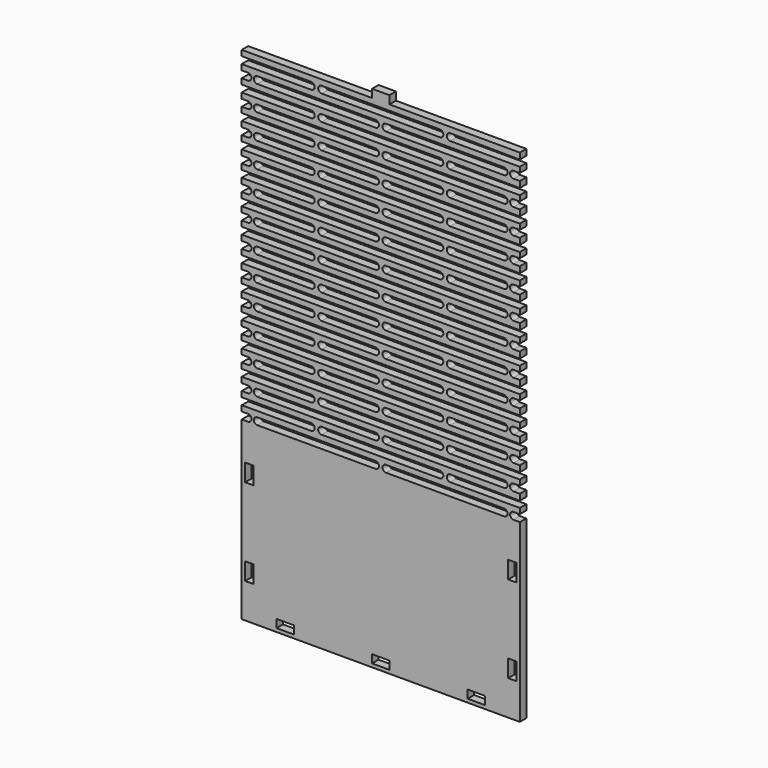
from build123d import *

# Parameters (mm, degrees)
F0_W     = 101.6
F0_H     = 63.5
F0_W_2   = 2.9718
F0_H_2   = 6.35
F0_W_3   = 6.35
F0_H_3   = 2.9718
F1_DEPTH = 2.9718


with BuildPart() as f1:
    # F0 (on Front) → F1 (new body)
    with BuildSketch(Plane.XZ):
        with Locations((0.0203015033, 4.5659675)):
            Rectangle(F0_W, F0_H)
        with Locations((-48.0237984967, -11.3090325)):
            Rectangle(F0_W_2, F0_H_2, mode=Mode.SUBTRACT)
        with Locations((-34.9046984967, -24.4281325)):
            Rectangle(F0_W_3, F0_H_3, mode=Mode.SUBTRACT)
        with Locations((0.0203015033, -24.4281325)):
            Rectangle(F0_W_3, F0_H_3, mode=Mode.SUBTRACT)
        with Locations((-48.0237984967, 20.4409675)):
            Rectangle(F0_W_2, F0_H_2, mode=Mode.SUBTRACT)
        with Locations((34.9453015033, -24.4281325)):
            Rectangle(F0_W_3, F0_H_3, mode=Mode.SUBTRACT)
        with Locations((48.0644015033, -11.3090325)):
            Rectangle(F0_W_2, F0_H_2, mode=Mode.SUBTRACT)
        with Locations((48.0644015033, 20.4409675)):
            Rectangle(F0_W_2, F0_H_2, mode=Mode.SUBTRACT)
        with BuildLine():
            Line((-50.7796984967, 36.3159675), (50.8203015033, 36.3159675))
            Line((50.8203015033, 36.3159675), (50.8203015033, 37.0779675))
            Line((50.8203015033, 37.0779675), (48.5343015033, 37.0779675))
            ThreePointArc((48.5343015033, 37.0779675), (47.2643015033, 38.3479675), (48.5343015033, 39.6179675))
            Line((48.5343015033, 39.6179675), (50.8203015033, 39.6179675))
            Line((50.8203015033, 39.6179675), (50.8203015033, 41.6499675))
            Line((50.8203015033, 41.6499675), (25.4192259187, 41.6502592084))
            ThreePointArc((25.4192259187, 41.6502592084), (24.1386144114, 42.9207526874), (25.4203015033, 44.1901610973))
            Line((25.4203015033, 44.1901610973), (50.8203015033, 43.956407084))
            Line((50.8203015033, 43.956407084), (50.8203015033, 46.2219675))
            Line((50.8203015033, 46.2219675), (48.5343015033, 46.2219675))
            ThreePointArc((48.5343015033, 46.2219675), (47.2643015033, 47.4919675), (48.5343015033, 48.7619675))
            Line((48.5343015033, 48.7619675), (50.8203015033, 48.7619675))
            Line((50.8203015033, 48.7619675), (50.8203015033, 50.7939675))
            Line((50.8203015033, 50.7939675), (25.4192259187, 50.7942592084))
            ThreePointArc((25.4192259187, 50.7942592084), (24.1386144114, 52.0647526874), (25.4203015033, 53.3341610973))
            Line((25.4203015033, 53.3341610973), (50.8203015033, 53.100407084))
            Line((50.8203015033, 53.100407084), (50.8203015033, 55.3659675))
            Line((50.8203015033, 55.3659675), (48.5343015033, 55.3659675))
            ThreePointArc((48.5343015033, 55.3659675), (47.2643015033, 56.6359675), (48.5343015033, 57.9059675))
            Line((48.5343015033, 57.9059675), (50.8203015033, 57.9059675))
            Line((50.8203015033, 57.9059675), (50.8203015033, 59.9379675))
            Line((50.8203015033, 59.9379675), (25.4192259187, 59.9382592084))
            ThreePointArc((25.4192259187, 59.9382592084), (24.1386144114, 61.2087526874), (25.4203015033, 62.4781610973))
            Line((25.4203015033, 62.4781610973), (50.8203015033, 62.244407084))
            Line((50.8203015033, 62.244407084), (50.8203015033, 64.5099675))
            Line((50.8203015033, 64.5099675), (48.5343015033, 64.5099675))
            ThreePointArc((48.5343015033, 64.5099675), (47.2643015033, 65.7799675), (48.5343015033, 67.0499675))
            Line((48.5343015033, 67.0499675), (50.8203015033, 67.0499675))
            Line((50.8203015033, 67.0499675), (50.8203015033, 69.0819675))
            Line((50.8203015033, 69.0819675), (25.4192259187, 69.0822592084))
            ThreePointArc((25.4192259187, 69.0822592084), (24.1386144114, 70.3527526874), (25.4203015033, 71.6221610973))
            Line((25.4203015033, 71.6221610973), (50.8203015033, 71.388407084))
            Line((50.8203015033, 71.388407084), (50.8203015033, 73.6539675))
            Line((50.8203015033, 73.6539675), (48.5343015033, 73.6539675))
            ThreePointArc((48.5343015033, 73.6539675), (47.2643015033, 74.9239675), (48.5343015033, 76.1939675))
            Line((48.5343015033, 76.1939675), (50.8203015033, 76.1939675))
            Line((50.8203015033, 76.1939675), (50.8203015033, 78.2259675))
            Line((50.8203015033, 78.2259675), (25.4192259187, 78.2262592084))
            ThreePointArc((25.4192259187, 78.2262592084), (24.1386144114, 79.4967526874), (25.4203015033, 80.7661610973))
            Line((25.4203015033, 80.7661610973), (50.8203015033, 80.532407084))
            Line((50.8203015033, 80.532407084), (50.8203015033, 82.7979675))
            Line((50.8203015033, 82.7979675), (48.5343015033, 82.7979675))
            ThreePointArc((48.5343015033, 82.7979675), (47.2643015033, 84.0679675), (48.5343015033, 85.3379675))
            Line((48.5343015033, 85.3379675), (50.8203015033, 85.3379675))
            Line((50.8203015033, 85.3379675), (50.8203015033, 87.3699675))
            Line((50.8203015033, 87.3699675), (25.4192259187, 87.3702592084))
            ThreePointArc((25.4192259187, 87.3702592084), (24.1386144114, 88.6407526874), (25.4203015033, 89.9101610973))
            Line((25.4203015033, 89.9101610973), (50.8203015033, 89.676407084))
            Line((50.8203015033, 89.676407084), (50.8203015033, 91.9419675))
            Line((50.8203015033, 91.9419675), (48.5343015033, 91.9419675))
            ThreePointArc((48.5343015033, 91.9419675), (47.2643015033, 93.2119675), (48.5343015033, 94.4819675))
            Line((48.5343015033, 94.4819675), (50.8203015033, 94.4819675))
            Line((50.8203015033, 94.4819675), (50.8203015033, 96.5139675))
            Line((50.8203015033, 96.5139675), (25.4192259187, 96.5142592084))
            ThreePointArc((25.4192259187, 96.5142592084), (24.1386144114, 97.7847526874), (25.4203015033, 99.0541610973))
            Line((25.4203015033, 99.0541610973), (50.8203015033, 98.820407084))
            Line((50.8203015033, 98.820407084), (50.8203015033, 101.0859675))
            Line((50.8203015033, 101.0859675), (48.5343015033, 101.0859675))
            ThreePointArc((48.5343015033, 101.0859675), (47.2643015033, 102.3559675), (48.5343015033, 103.6259675))
            Line((48.5343015033, 103.6259675), (50.8203015033, 103.6259675))
            Line((50.8203015033, 103.6259675), (50.8203015033, 105.6579675))
            Line((50.8203015033, 105.6579675), (25.4192259187, 105.6582592084))
            ThreePointArc((25.4192259187, 105.6582592084), (24.1386144114, 106.9287526874), (25.4203015033, 108.1981610973))
            Line((25.4203015033, 108.1981610973), (50.8203015033, 107.964407084))
            Line((50.8203015033, 107.964407084), (50.8203015033, 110.2299675))
            Line((50.8203015033, 110.2299675), (48.5343015033, 110.2299675))
            ThreePointArc((48.5343015033, 110.2299675), (47.2643015033, 111.4999675), (48.5343015033, 112.7699675))
            Line((48.5343015033, 112.7699675), (50.8203015033, 112.7699675))
            Line((50.8203015033, 112.7699675), (50.8203015033, 114.8019675))
            Line((50.8203015033, 114.8019675), (25.4192259187, 114.8022592084))
            ThreePointArc((25.4192259187, 114.8022592084), (24.1386144114, 116.0727526874), (25.4203015033, 117.3421610973))
            Line((25.4203015033, 117.3421610973), (50.8203015033, 117.108407084))
            Line((50.8203015033, 117.108407084), (50.8203015033, 119.3739675))
            Line((50.8203015033, 119.3739675), (48.5343015033, 119.3739675))
            ThreePointArc((48.5343015033, 119.3739675), (47.2643015033, 120.6439675), (48.5343015033, 121.9139675))
            Line((48.5343015033, 121.9139675), (50.8203015033, 121.9139675))
            Line((50.8203015033, 121.9139675), (50.8203015033, 123.9459675))
            Line((50.8203015033, 123.9459675), (25.4192259187, 123.9462592084))
            ThreePointArc((25.4192259187, 123.9462592084), (24.1386144114, 125.2167526874), (25.4203015033, 126.4861610973))
            Line((25.4203015033, 126.4861610973), (50.8203015033, 126.252407084))
            Line((50.8203015033, 126.252407084), (50.8203015033, 128.5179675))
            Line((50.8203015033, 128.5179675), (48.5343015033, 128.5179675))
            ThreePointArc((48.5343015033, 128.5179675), (47.2643015033, 129.7879675), (48.5343015033, 131.0579675))
            Line((48.5343015033, 131.0579675), (50.8203015033, 131.0579675))
            Line((50.8203015033, 131.0579675), (50.8203015033, 133.0899675))
            Line((50.8203015033, 133.0899675), (25.4192259187, 133.0902592084))
            ThreePointArc((25.4192259187, 133.0902592084), (24.1386144114, 134.3607526874), (25.4203015033, 135.6301610973))
            Line((25.4203015033, 135.6301610973), (50.8203015033, 135.396407084))
            Line((50.8203015033, 135.396407084), (50.8203015033, 137.6619675))
            Line((50.8203015033, 137.6619675), (48.5343015033, 137.6619675))
            ThreePointArc((48.5343015033, 137.6619675), (47.2643015033, 138.9319675), (48.5343015033, 140.2019675))
            Line((48.5343015033, 140.2019675), (50.8203015033, 140.2019675))
            Line((50.8203015033, 140.2019675), (50.8203015033, 142.2339675))
            Line((50.8203015033, 142.2339675), (25.4192259187, 142.2342592084))
            ThreePointArc((25.4192259187, 142.2342592084), (24.1386144114, 143.5047526874), (25.4203015033, 144.7741610973))
            Line((25.4203015033, 144.7741610973), (50.8203015033, 144.540407084))
            Line((50.8203015033, 144.540407084), (50.8203015033, 146.8059675))
            Line((50.8203015033, 146.8059675), (48.5343015033, 146.8059675))
            ThreePointArc((48.5343015033, 146.8059675), (47.2643015033, 148.0759675), (48.5343015033, 149.3459675))
            Line((48.5343015033, 149.3459675), (50.8203015033, 149.3459675))
            Line((50.8203015033, 149.3459675), (50.8203015033, 151.3779675))
            Line((50.8203015033, 151.3779675), (25.4192259187, 151.3782592084))
            ThreePointArc((25.4192259187, 151.3782592084), (24.1386144114, 152.6487526874), (25.4203015033, 153.9181610973))
            Line((25.4203015033, 153.9181610973), (50.8203015033, 153.684407084))
            Line((50.8203015033, 153.684407084), (50.8203015033, 155.9499675))
            Line((50.8203015033, 155.9499675), (3.1953015033, 155.9499675))
            Line((3.1953015033, 155.9499675), (-3.1546984967, 155.9499675))
            Line((-3.1546984967, 155.9499675), (-50.7796984967, 155.9499675))
            Line((-50.7796984967, 155.9499675), (-50.7796984967, 153.9179675))
            Line((-50.7796984967, 153.9179675), (-25.3796984967, 153.9179675))
            ThreePointArc((-25.3796984967, 153.9179675), (-24.1096984967, 152.6479675), (-25.3796984967, 151.3779675))
            Line((-25.3796984967, 151.3779675), (-50.7796984967, 151.3779675))
            Line((-50.7796984967, 151.3779675), (-50.7796984967, 149.3459675))
            Line((-50.7796984967, 149.3459675), (-48.4936984967, 149.3459675))
            ThreePointArc((-48.4936984967, 149.3459675), (-47.2236984967, 148.0759675), (-48.4936984967, 146.8059675))
            Line((-48.4936984967, 146.8059675), (-50.7796984967, 146.8059675))
            Line((-50.7796984967, 146.8059675), (-50.7796984967, 144.7739675))
            Line((-50.7796984967, 144.7739675), (-25.3796984967, 144.7739675))
            ThreePointArc((-25.3796984967, 144.7739675), (-24.1096984967, 143.5039675), (-25.3796984967, 142.2339675))
            Line((-25.3796984967, 142.2339675), (-50.7796984967, 142.2339675))
            Line((-50.7796984967, 142.2339675), (-50.7796984967, 140.2019675))
            Line((-50.7796984967, 140.2019675), (-48.4936984967, 140.2019675))
            ThreePointArc((-48.4936984967, 140.2019675), (-47.2236984967, 138.9319675), (-48.4936984967, 137.6619675))
            Line((-48.4936984967, 137.6619675), (-50.7796984967, 137.6619675))
            Line((-50.7796984967, 137.6619675), (-50.7796984967, 135.6299675))
            Line((-50.7796984967, 135.6299675), (-25.3796984967, 135.6299675))
            ThreePointArc((-25.3796984967, 135.6299675), (-24.1096984967, 134.3599675), (-25.3796984967, 133.0899675))
            Line((-25.3796984967, 133.0899675), (-50.7796984967, 133.0899675))
            Line((-50.7796984967, 133.0899675), (-50.7796984967, 131.0579675))
            Line((-50.7796984967, 131.0579675), (-48.4936984967, 131.0579675))
            ThreePointArc((-48.4936984967, 131.0579675), (-47.2236984967, 129.7879675), (-48.4936984967, 128.5179675))
            Line((-48.4936984967, 128.5179675), (-50.7796984967, 128.5179675))
            Line((-50.7796984967, 128.5179675), (-50.7796984967, 126.4859675))
            Line((-50.7796984967, 126.4859675), (-25.3796984967, 126.4859675))
            ThreePointArc((-25.3796984967, 126.4859675), (-24.1096984967, 125.2159675), (-25.3796984967, 123.9459675))
            Line((-25.3796984967, 123.9459675), (-50.7796984967, 123.9459675))
            Line((-50.7796984967, 123.9459675), (-50.7796984967, 121.9139675))
            Line((-50.7796984967, 121.9139675), (-48.4936984967, 121.9139675))
            ThreePointArc((-48.4936984967, 121.9139675), (-47.2236984967, 120.6439675), (-48.4936984967, 119.3739675))
            Line((-48.4936984967, 119.3739675), (-50.7796984967, 119.3739675))
            Line((-50.7796984967, 119.3739675), (-50.7796984967, 117.3419675))
            Line((-50.7796984967, 117.3419675), (-25.3796984967, 117.3419675))
            ThreePointArc((-25.3796984967, 117.3419675), (-24.1096984967, 116.0719675), (-25.3796984967, 114.8019675))
            Line((-25.3796984967, 114.8019675), (-50.7796984967, 114.8019675))
            Line((-50.7796984967, 114.8019675), (-50.7796984967, 112.7699675))
            Line((-50.7796984967, 112.7699675), (-48.4936984967, 112.7699675))
            ThreePointArc((-48.4936984967, 112.7699675), (-47.2236984967, 111.4999675), (-48.4936984967, 110.2299675))
            Line((-48.4936984967, 110.2299675), (-50.7796984967, 110.2299675))
            Line((-50.7796984967, 110.2299675), (-50.7796984967, 108.1979675))
            Line((-50.7796984967, 108.1979675), (-25.3796984967, 108.1979675))
            ThreePointArc((-25.3796984967, 108.1979675), (-24.1096984967, 106.9279675), (-25.3796984967, 105.6579675))
            Line((-25.3796984967, 105.6579675), (-50.7796984967, 105.6579675))
            Line((-50.7796984967, 105.6579675), (-50.7796984967, 103.6259675))
            Line((-50.7796984967, 103.6259675), (-48.4936984967, 103.6259675))
            ThreePointArc((-48.4936984967, 103.6259675), (-47.2236984967, 102.3559675), (-48.4936984967, 101.0859675))
            Line((-48.4936984967, 101.0859675), (-50.7796984967, 101.0859675))
            Line((-50.7796984967, 101.0859675), (-50.7796984967, 99.0539675))
            Line((-50.7796984967, 99.0539675), (-25.3796984967, 99.0539675))
            ThreePointArc((-25.3796984967, 99.0539675), (-24.1096984967, 97.7839675), (-25.3796984967, 96.5139675))
            Line((-25.3796984967, 96.5139675), (-50.7796984967, 96.5139675))
            Line((-50.7796984967, 96.5139675), (-50.7796984967, 94.4819675))
            Line((-50.7796984967, 94.4819675), (-48.4936984967, 94.4819675))
            ThreePointArc((-48.4936984967, 94.4819675), (-47.2236984967, 93.2119675), (-48.4936984967, 91.9419675))
            Line((-48.4936984967, 91.9419675), (-50.7796984967, 91.9419675))
            Line((-50.7796984967, 91.9419675), (-50.7796984967, 89.9099675))
            Line((-50.7796984967, 89.9099675), (-25.3796984967, 89.9099675))
            ThreePointArc((-25.3796984967, 89.9099675), (-24.1096984967, 88.6399675), (-25.3796984967, 87.3699675))
            Line((-25.3796984967, 87.3699675), (-50.7796984967, 87.3699675))
            Line((-50.7796984967, 87.3699675), (-50.7796984967, 85.3379675))
            Line((-50.7796984967, 85.3379675), (-48.4936984967, 85.3379675))
            ThreePointArc((-48.4936984967, 85.3379675), (-47.2236984967, 84.0679675), (-48.4936984967, 82.7979675))
            Line((-48.4936984967, 82.7979675), (-50.7796984967, 82.7979675))
            Line((-50.7796984967, 82.7979675), (-50.7796984967, 80.7659675))
            Line((-50.7796984967, 80.7659675), (-25.3796984967, 80.7659675))
            ThreePointArc((-25.3796984967, 80.7659675), (-24.1096984967, 79.4959675), (-25.3796984967, 78.2259675))
            Line((-25.3796984967, 78.2259675), (-50.7796984967, 78.2259675))
            Line((-50.7796984967, 78.2259675), (-50.7796984967, 76.1939675))
            Line((-50.7796984967, 76.1939675), (-48.4936984967, 76.1939675))
            ThreePointArc((-48.4936984967, 76.1939675), (-47.2236984967, 74.9239675), (-48.4936984967, 73.6539675))
            Line((-48.4936984967, 73.6539675), (-50.7796984967, 73.6539675))
            Line((-50.7796984967, 73.6539675), (-50.7796984967, 71.6219675))
            Line((-50.7796984967, 71.6219675), (-25.3796984967, 71.6219675))
            ThreePointArc((-25.3796984967, 71.6219675), (-24.1096984967, 70.3519675), (-25.3796984967, 69.0819675))
            Line((-25.3796984967, 69.0819675), (-50.7796984967, 69.0819675))
            Line((-50.7796984967, 69.0819675), (-50.7796984967, 67.0499675))
            Line((-50.7796984967, 67.0499675), (-48.4936984967, 67.0499675))
            ThreePointArc((-48.4936984967, 67.0499675), (-47.2236984967, 65.7799675), (-48.4936984967, 64.5099675))
            Line((-48.4936984967, 64.5099675), (-50.7796984967, 64.5099675))
            Line((-50.7796984967, 64.5099675), (-50.7796984967, 62.4779675))
            Line((-50.7796984967, 62.4779675), (-25.3796984967, 62.4779675))
            ThreePointArc((-25.3796984967, 62.4779675), (-24.1096984967, 61.2079675), (-25.3796984967, 59.9379675))
            Line((-25.3796984967, 59.9379675), (-50.7796984967, 59.9379675))
            Line((-50.7796984967, 59.9379675), (-50.7796984967, 57.9059675))
            Line((-50.7796984967, 57.9059675), (-48.4936984967, 57.9059675))
            ThreePointArc((-48.4936984967, 57.9059675), (-47.2236984967, 56.6359675), (-48.4936984967, 55.3659675))
            Line((-48.4936984967, 55.3659675), (-50.7796984967, 55.3659675))
            Line((-50.7796984967, 55.3659675), (-50.7796984967, 53.3339675))
            Line((-50.7796984967, 53.3339675), (-25.3796984967, 53.3339675))
            ThreePointArc((-25.3796984967, 53.3339675), (-24.1096984967, 52.0639675), (-25.3796984967, 50.7939675))
            Line((-25.3796984967, 50.7939675), (-50.7796984967, 50.7939675))
            Line((-50.7796984967, 50.7939675), (-50.7796984967, 48.7619675))
            Line((-50.7796984967, 48.7619675), (-48.4936984967, 48.7619675))
            ThreePointArc((-48.4936984967, 48.7619675), (-47.2236984967, 47.4919675), (-48.4936984967, 46.2219675))
            Line((-48.4936984967, 46.2219675), (-50.7796984967, 46.2219675))
            Line((-50.7796984967, 46.2219675), (-50.7796984967, 44.1899675))
            Line((-50.7796984967, 44.1899675), (-25.3796984967, 44.1899675))
            ThreePointArc((-25.3796984967, 44.1899675), (-24.1096984967, 42.9199675), (-25.3796984967, 41.6499675))
            Line((-25.3796984967, 41.6499675), (-50.7796984967, 41.6499675))
            Line((-50.7796984967, 41.6499675), (-50.7796984967, 39.6179675))
            Line((-50.7796984967, 39.6179675), (-48.4936984967, 39.6179675))
            ThreePointArc((-48.4936984967, 39.6179675), (-47.2236984967, 38.3479675), (-48.4936984967, 37.0779675))
            Line((-48.4936984967, 37.0779675), (-50.7796984967, 37.0779675))
            Line((-50.7796984967, 37.0779675), (-50.7796984967, 36.3159675))
        make_face()
        with BuildLine():
            Line((-45.0646984967, 39.6179675), (-1.8846984967, 39.6179675))
            ThreePointArc((-1.8846984967, 39.6179675), (-0.6146984967, 38.3479675), (-1.8846984967, 37.0779675))
            Line((-1.8846984967, 37.0779675), (-45.0646984967, 37.0779675))
            ThreePointArc((-45.0646984967, 37.0779675), (-46.3346984967, 38.3479675), (-45.0646984967, 39.6179675))
        make_face(mode=Mode.SUBTRACT)
        with BuildLine():
            Line((-45.0646984967, 48.7619675), (-1.8846984967, 48.7619675))
            ThreePointArc((-1.8846984967, 48.7619675), (-0.6146984967, 47.4919675), (-1.8846984967, 46.2219675))
            Line((-1.8846984967, 46.2219675), (-45.0646984967, 46.2219675))
            ThreePointArc((-45.0646984967, 46.2219675), (-46.3346984967, 47.4919675), (-45.0646984967, 48.7619675))
        make_face(mode=Mode.SUBTRACT)
        with BuildLine():
            Line((-45.0646984967, 57.9059675), (-1.8846984967, 57.9059675))
            ThreePointArc((-1.8846984967, 57.9059675), (-0.6146984967, 56.6359675), (-1.8846984967, 55.3659675))
            Line((-1.8846984967, 55.3659675), (-45.0646984967, 55.3659675))
            ThreePointArc((-45.0646984967, 55.3659675), (-46.3346984967, 56.6359675), (-45.0646984967, 57.9059675))
        make_face(mode=Mode.SUBTRACT)
        with BuildLine():
            Line((-45.0646984967, 67.0499675), (-1.8846984967, 67.0499675))
            ThreePointArc((-1.8846984967, 67.0499675), (-0.6146984967, 65.7799675), (-1.8846984967, 64.5099675))
            Line((-1.8846984967, 64.5099675), (-45.0646984967, 64.5099675))
            ThreePointArc((-45.0646984967, 64.5099675), (-46.3346984967, 65.7799675), (-45.0646984967, 67.0499675))
        make_face(mode=Mode.SUBTRACT)
        with BuildLine():
            ThreePointArc((-21.5696984967, 41.6499675), (-22.8397092794, 42.9199782827), (-21.5696984967, 44.1899890654))
            Line((-21.5696984967, 44.1899890654), (21.6103015033, 44.1899890654))
            ThreePointArc((21.6103015033, 44.1899890654), (22.880312286, 42.9199782827), (21.6103015033, 41.6499675))
            Line((21.6103015033, 41.6499675), (-21.5696984967, 41.6499675))
        make_face(mode=Mode.SUBTRACT)
        with BuildLine():
            ThreePointArc((-21.5696984967, 50.7939675), (-22.8397092794, 52.0639782827), (-21.5696984967, 53.3339890654))
            Line((-21.5696984967, 53.3339890654), (21.6103015033, 53.3339890654))
            ThreePointArc((21.6103015033, 53.3339890654), (22.880312286, 52.0639782827), (21.6103015033, 50.7939675))
            Line((21.6103015033, 50.7939675), (-21.5696984967, 50.7939675))
        make_face(mode=Mode.SUBTRACT)
        with BuildLine():
            ThreePointArc((-21.5696984967, 59.9379675), (-22.8397092794, 61.2079782827), (-21.5696984967, 62.4779890654))
            Line((-21.5696984967, 62.4779890654), (21.6103015033, 62.4779890654))
            ThreePointArc((21.6103015033, 62.4779890654), (22.880312286, 61.2079782827), (21.6103015033, 59.9379675))
            Line((21.6103015033, 59.9379675), (-21.5696984967, 59.9379675))
        make_face(mode=Mode.SUBTRACT)
        with BuildLine():
            Line((1.9253015033, 39.6179675), (45.1053015033, 39.6179675))
            ThreePointArc((45.1053015033, 39.6179675), (46.3753015033, 38.3479675), (45.1053015033, 37.0779675))
            Line((45.1053015033, 37.0779675), (1.9253015033, 37.0779675))
            ThreePointArc((1.9253015033, 37.0779675), (0.6553015033, 38.3479675), (1.9253015033, 39.6179675))
        make_face(mode=Mode.SUBTRACT)
        with BuildLine():
            Line((1.9253015033, 48.7619675), (45.1053015033, 48.7619675))
            ThreePointArc((45.1053015033, 48.7619675), (46.3753015033, 47.4919675), (45.1053015033, 46.2219675))
            Line((45.1053015033, 46.2219675), (1.9253015033, 46.2219675))
            ThreePointArc((1.9253015033, 46.2219675), (0.6553015033, 47.4919675), (1.9253015033, 48.7619675))
        make_face(mode=Mode.SUBTRACT)
        with BuildLine():
            Line((1.9253015033, 57.9059675), (45.1053015033, 57.9059675))
            ThreePointArc((45.1053015033, 57.9059675), (46.3753015033, 56.6359675), (45.1053015033, 55.3659675))
            Line((45.1053015033, 55.3659675), (1.9253015033, 55.3659675))
            ThreePointArc((1.9253015033, 55.3659675), (0.6553015033, 56.6359675), (1.9253015033, 57.9059675))
        make_face(mode=Mode.SUBTRACT)
        with BuildLine():
            Line((1.9253015033, 67.0499675), (45.1053015033, 67.0499675))
            ThreePointArc((45.1053015033, 67.0499675), (46.3753015033, 65.7799675), (45.1053015033, 64.5099675))
            Line((45.1053015033, 64.5099675), (1.9253015033, 64.5099675))
            ThreePointArc((1.9253015033, 64.5099675), (0.6553015033, 65.7799675), (1.9253015033, 67.0499675))
        make_face(mode=Mode.SUBTRACT)
        with BuildLine():
            Line((-45.0646984967, 76.1939675), (-1.8846984967, 76.1939675))
            ThreePointArc((-1.8846984967, 76.1939675), (-0.6146984967, 74.9239675), (-1.8846984967, 73.6539675))
            Line((-1.8846984967, 73.6539675), (-45.0646984967, 73.6539675))
            ThreePointArc((-45.0646984967, 73.6539675), (-46.3346984967, 74.9239675), (-45.0646984967, 76.1939675))
        make_face(mode=Mode.SUBTRACT)
        with BuildLine():
            Line((-45.0646984967, 85.3379675), (-1.8846984967, 85.3379675))
            ThreePointArc((-1.8846984967, 85.3379675), (-0.6146984967, 84.0679675), (-1.8846984967, 82.7979675))
            Line((-1.8846984967, 82.7979675), (-45.0646984967, 82.7979675))
            ThreePointArc((-45.0646984967, 82.7979675), (-46.3346984967, 84.0679675), (-45.0646984967, 85.3379675))
        make_face(mode=Mode.SUBTRACT)
        with BuildLine():
            ThreePointArc((-21.5696984967, 69.0819675), (-22.8397092794, 70.3519782827), (-21.5696984967, 71.6219890654))
            Line((-21.5696984967, 71.6219890654), (21.6103015033, 71.6219890654))
            ThreePointArc((21.6103015033, 71.6219890654), (22.880312286, 70.3519782827), (21.6103015033, 69.0819675))
            Line((21.6103015033, 69.0819675), (-21.5696984967, 69.0819675))
        make_face(mode=Mode.SUBTRACT)
        with BuildLine():
            ThreePointArc((-21.5696984967, 78.2259675), (-22.8397092794, 79.4959782827), (-21.5696984967, 80.7659890654))
            Line((-21.5696984967, 80.7659890654), (21.6103015033, 80.7659890654))
            ThreePointArc((21.6103015033, 80.7659890654), (22.880312286, 79.4959782827), (21.6103015033, 78.2259675))
            Line((21.6103015033, 78.2259675), (-21.5696984967, 78.2259675))
        make_face(mode=Mode.SUBTRACT)
        with BuildLine():
            ThreePointArc((-21.5696984967, 87.3699675), (-22.8397092794, 88.6399782827), (-21.5696984967, 89.9099890654))
            Line((-21.5696984967, 89.9099890654), (21.6103015033, 89.9099890654))
            ThreePointArc((21.6103015033, 89.9099890654), (22.880312286, 88.6399782827), (21.6103015033, 87.3699675))
            Line((21.6103015033, 87.3699675), (-21.5696984967, 87.3699675))
        make_face(mode=Mode.SUBTRACT)
        with BuildLine():
            Line((-45.0646984967, 94.4819675), (-1.8846984967, 94.4819675))
            ThreePointArc((-1.8846984967, 94.4819675), (-0.6146984967, 93.2119675), (-1.8846984967, 91.9419675))
            Line((-1.8846984967, 91.9419675), (-45.0646984967, 91.9419675))
            ThreePointArc((-45.0646984967, 91.9419675), (-46.3346984967, 93.2119675), (-45.0646984967, 94.4819675))
        make_face(mode=Mode.SUBTRACT)
        with BuildLine():
            Line((-45.0646984967, 103.6259675), (-1.8846984967, 103.6259675))
            ThreePointArc((-1.8846984967, 103.6259675), (-0.6146984967, 102.3559675), (-1.8846984967, 101.0859675))
            Line((-1.8846984967, 101.0859675), (-45.0646984967, 101.0859675))
            ThreePointArc((-45.0646984967, 101.0859675), (-46.3346984967, 102.3559675), (-45.0646984967, 103.6259675))
        make_face(mode=Mode.SUBTRACT)
        with BuildLine():
            Line((-45.0646984967, 112.7699675), (-1.8846984967, 112.7699675))
            ThreePointArc((-1.8846984967, 112.7699675), (-0.6146984967, 111.4999675), (-1.8846984967, 110.2299675))
            Line((-1.8846984967, 110.2299675), (-45.0646984967, 110.2299675))
            ThreePointArc((-45.0646984967, 110.2299675), (-46.3346984967, 111.4999675), (-45.0646984967, 112.7699675))
        make_face(mode=Mode.SUBTRACT)
        with BuildLine():
            ThreePointArc((-21.5696984967, 96.5139675), (-22.8397092794, 97.7839782827), (-21.5696984967, 99.0539890654))
            Line((-21.5696984967, 99.0539890654), (21.6103015033, 99.0539890654))
            ThreePointArc((21.6103015033, 99.0539890654), (22.880312286, 97.7839782827), (21.6103015033, 96.5139675))
            Line((21.6103015033, 96.5139675), (-21.5696984967, 96.5139675))
        make_face(mode=Mode.SUBTRACT)
        with BuildLine():
            ThreePointArc((-21.5696984967, 105.6579675), (-22.8397092794, 106.9279782827), (-21.5696984967, 108.1979890654))
            Line((-21.5696984967, 108.1979890654), (21.6103015033, 108.1979890654))
            ThreePointArc((21.6103015033, 108.1979890654), (22.880312286, 106.9279782827), (21.6103015033, 105.6579675))
            Line((21.6103015033, 105.6579675), (-21.5696984967, 105.6579675))
        make_face(mode=Mode.SUBTRACT)
        with BuildLine():
            Line((-45.0646984967, 121.9139675), (-1.8846984967, 121.9139675))
            ThreePointArc((-1.8846984967, 121.9139675), (-0.6146984967, 120.6439675), (-1.8846984967, 119.3739675))
            Line((-1.8846984967, 119.3739675), (-45.0646984967, 119.3739675))
            ThreePointArc((-45.0646984967, 119.3739675), (-46.3346984967, 120.6439675), (-45.0646984967, 121.9139675))
        make_face(mode=Mode.SUBTRACT)
        with BuildLine():
            Line((-45.0646984967, 131.0579675), (-1.8846984967, 131.0579675))
            ThreePointArc((-1.8846984967, 131.0579675), (-0.6146984967, 129.7879675), (-1.8846984967, 128.5179675))
            Line((-1.8846984967, 128.5179675), (-45.0646984967, 128.5179675))
            ThreePointArc((-45.0646984967, 128.5179675), (-46.3346984967, 129.7879675), (-45.0646984967, 131.0579675))
        make_face(mode=Mode.SUBTRACT)
        with BuildLine():
            ThreePointArc((-21.5696984967, 114.8019675), (-22.8397092794, 116.0719782827), (-21.5696984967, 117.3419890654))
            Line((-21.5696984967, 117.3419890654), (21.6103015033, 117.3419890654))
            ThreePointArc((21.6103015033, 117.3419890654), (22.880312286, 116.0719782827), (21.6103015033, 114.8019675))
            Line((21.6103015033, 114.8019675), (-21.5696984967, 114.8019675))
        make_face(mode=Mode.SUBTRACT)
        with BuildLine():
            ThreePointArc((-21.5696984967, 123.9459675), (-22.8397092794, 125.2159782827), (-21.5696984967, 126.4859890654))
            Line((-21.5696984967, 126.4859890654), (21.6103015033, 126.4859890654))
            ThreePointArc((21.6103015033, 126.4859890654), (22.880312286, 125.2159782827), (21.6103015033, 123.9459675))
            Line((21.6103015033, 123.9459675), (-21.5696984967, 123.9459675))
        make_face(mode=Mode.SUBTRACT)
        with BuildLine():
            ThreePointArc((-21.5696984967, 133.0899675), (-22.8397092794, 134.3599782827), (-21.5696984967, 135.6299890654))
            Line((-21.5696984967, 135.6299890654), (21.6103015033, 135.6299890654))
            ThreePointArc((21.6103015033, 135.6299890654), (22.880312286, 134.3599782827), (21.6103015033, 133.0899675))
            Line((21.6103015033, 133.0899675), (-21.5696984967, 133.0899675))
        make_face(mode=Mode.SUBTRACT)
        with BuildLine():
            Line((-45.0646984967, 140.2019675), (-1.8846984967, 140.2019675))
            ThreePointArc((-1.8846984967, 140.2019675), (-0.6146984967, 138.9319675), (-1.8846984967, 137.6619675))
            Line((-1.8846984967, 137.6619675), (-45.0646984967, 137.6619675))
            ThreePointArc((-45.0646984967, 137.6619675), (-46.3346984967, 138.9319675), (-45.0646984967, 140.2019675))
        make_face(mode=Mode.SUBTRACT)
        with BuildLine():
            ThreePointArc((-45.0646984967, 146.8059675), (-46.3346984967, 148.0759675), (-45.0646984967, 149.3459675))
            Line((-45.0646984967, 149.3459675), (-1.8846984967, 149.3459675))
            ThreePointArc((-1.8846984967, 149.3459675), (-0.6146984967, 148.0759675), (-1.8846984967, 146.8059675))
            Line((-1.8846984967, 146.8059675), (-45.0646984967, 146.8059675))
        make_face(mode=Mode.SUBTRACT)
        with BuildLine():
            ThreePointArc((-21.5696984967, 142.2339675), (-22.8397092794, 143.5039782827), (-21.5696984967, 144.7739890654))
            Line((-21.5696984967, 144.7739890654), (21.6103015033, 144.7739890654))
            ThreePointArc((21.6103015033, 144.7739890654), (22.880312286, 143.5039782827), (21.6103015033, 142.2339675))
            Line((21.6103015033, 142.2339675), (-21.5696984967, 142.2339675))
        make_face(mode=Mode.SUBTRACT)
        with BuildLine():
            ThreePointArc((-21.5696984967, 151.3779675), (-22.8397092794, 152.6479782827), (-21.5696984967, 153.9179890654))
            Line((-21.5696984967, 153.9179890654), (21.6103015033, 153.9179890654))
            ThreePointArc((21.6103015033, 153.9179890654), (22.880312286, 152.6479782827), (21.6103015033, 151.3779675))
            Line((21.6103015033, 151.3779675), (-21.5696984967, 151.3779675))
        make_face(mode=Mode.SUBTRACT)
        with BuildLine():
            Line((1.9253015033, 76.1939675), (45.1053015033, 76.1939675))
            ThreePointArc((45.1053015033, 76.1939675), (46.3753015033, 74.9239675), (45.1053015033, 73.6539675))
            Line((45.1053015033, 73.6539675), (1.9253015033, 73.6539675))
            ThreePointArc((1.9253015033, 73.6539675), (0.6553015033, 74.9239675), (1.9253015033, 76.1939675))
        make_face(mode=Mode.SUBTRACT)
        with BuildLine():
            Line((1.9253015033, 85.3379675), (45.1053015033, 85.3379675))
            ThreePointArc((45.1053015033, 85.3379675), (46.3753015033, 84.0679675), (45.1053015033, 82.7979675))
            Line((45.1053015033, 82.7979675), (1.9253015033, 82.7979675))
            ThreePointArc((1.9253015033, 82.7979675), (0.6553015033, 84.0679675), (1.9253015033, 85.3379675))
        make_face(mode=Mode.SUBTRACT)
        with BuildLine():
            Line((1.9253015033, 94.4819675), (45.1053015033, 94.4819675))
            ThreePointArc((45.1053015033, 94.4819675), (46.3753015033, 93.2119675), (45.1053015033, 91.9419675))
            Line((45.1053015033, 91.9419675), (1.9253015033, 91.9419675))
            ThreePointArc((1.9253015033, 91.9419675), (0.6553015033, 93.2119675), (1.9253015033, 94.4819675))
        make_face(mode=Mode.SUBTRACT)
        with BuildLine():
            Line((1.9253015033, 103.6259675), (45.1053015033, 103.6259675))
            ThreePointArc((45.1053015033, 103.6259675), (46.3753015033, 102.3559675), (45.1053015033, 101.0859675))
            Line((45.1053015033, 101.0859675), (1.9253015033, 101.0859675))
            ThreePointArc((1.9253015033, 101.0859675), (0.6553015033, 102.3559675), (1.9253015033, 103.6259675))
        make_face(mode=Mode.SUBTRACT)
        with BuildLine():
            Line((1.9253015033, 112.7699675), (45.1053015033, 112.7699675))
            ThreePointArc((45.1053015033, 112.7699675), (46.3753015033, 111.4999675), (45.1053015033, 110.2299675))
            Line((45.1053015033, 110.2299675), (1.9253015033, 110.2299675))
            ThreePointArc((1.9253015033, 110.2299675), (0.6553015033, 111.4999675), (1.9253015033, 112.7699675))
        make_face(mode=Mode.SUBTRACT)
        with BuildLine():
            Line((1.9253015033, 121.9139675), (45.1053015033, 121.9139675))
            ThreePointArc((45.1053015033, 121.9139675), (46.3753015033, 120.6439675), (45.1053015033, 119.3739675))
            Line((45.1053015033, 119.3739675), (1.9253015033, 119.3739675))
            ThreePointArc((1.9253015033, 119.3739675), (0.6553015033, 120.6439675), (1.9253015033, 121.9139675))
        make_face(mode=Mode.SUBTRACT)
        with BuildLine():
            Line((1.9253015033, 131.0579675), (45.1053015033, 131.0579675))
            ThreePointArc((45.1053015033, 131.0579675), (46.3753015033, 129.7879675), (45.1053015033, 128.5179675))
            Line((45.1053015033, 128.5179675), (1.9253015033, 128.5179675))
            ThreePointArc((1.9253015033, 128.5179675), (0.6553015033, 129.7879675), (1.9253015033, 131.0579675))
        make_face(mode=Mode.SUBTRACT)
        with BuildLine():
            Line((1.9253015033, 140.2019675), (45.1053015033, 140.2019675))
            ThreePointArc((45.1053015033, 140.2019675), (46.3753015033, 138.9319675), (45.1053015033, 137.6619675))
            Line((45.1053015033, 137.6619675), (1.9253015033, 137.6619675))
            ThreePointArc((1.9253015033, 137.6619675), (0.6553015033, 138.9319675), (1.9253015033, 140.2019675))
        make_face(mode=Mode.SUBTRACT)
        with BuildLine():
            ThreePointArc((1.9253015033, 146.8059675), (0.6553015033, 148.0759675), (1.9253015033, 149.3459675))
            Line((1.9253015033, 149.3459675), (45.1053015033, 149.3459675))
            ThreePointArc((45.1053015033, 149.3459675), (46.3753015033, 148.0759675), (45.1053015033, 146.8059675))
            Line((45.1053015033, 146.8059675), (1.9253015033, 146.8059675))
        make_face(mode=Mode.SUBTRACT)
        with Locations((0.0203015033, 157.4358675)):
            Rectangle(F0_W_3, F0_H_3)
    extrude(amount=F1_DEPTH)


solid = f1.part
